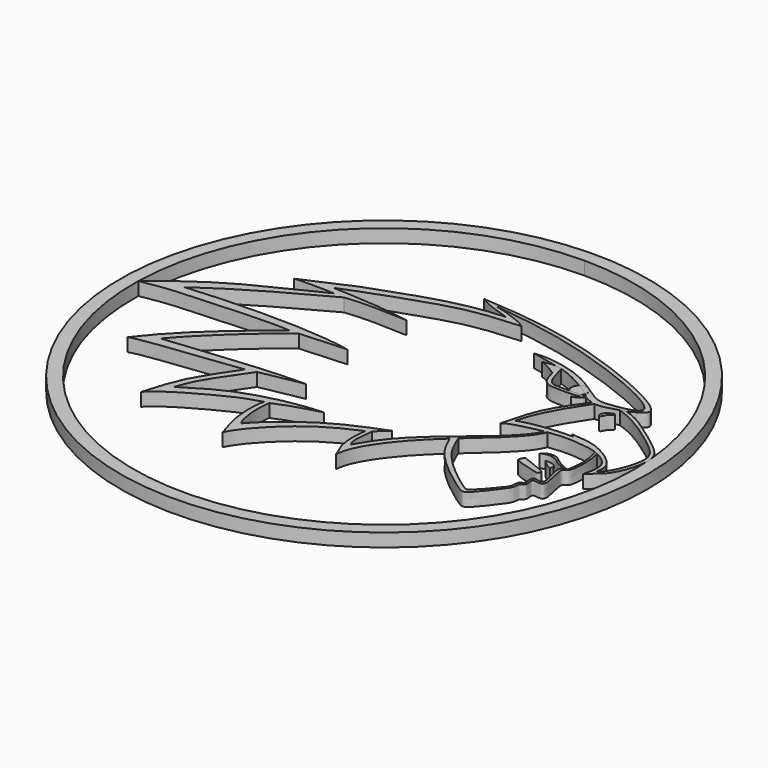
from build123d import *

# Parameters (mm, degrees)
F0_R     = 20
F1_DEPTH = 1
F3_DEPTH = 1
F4_DEPTH = 1
F5_DEPTH = 1


with BuildPart() as f1:
    # F0 (on Top) → F1 (new body)
    with BuildSketch(Plane.XY):
        Circle(F0_R)
        with BuildLine():
            ThreePointArc((0, 19), (13.4350288425, 13.4350288425), (19, 0))
            ThreePointArc((19, 0), (-13.4350288425, -13.4350288425), (0, 19))
        make_face(mode=Mode.SUBTRACT)
    extrude(amount=F1_DEPTH)

    # F0 (on Top) → F5 (cut)
    with BuildSketch(Plane.XY):
        with BuildLine():
            ThreePointArc((2, 17), (1.4142135624, 18.4142135624), (0, 19))
            ThreePointArc((0, 19), (-1.4142135624, 15.5857864376), (2, 17))
        make_face()
    extrude(amount=-F5_DEPTH, mode=Mode.SUBTRACT)


with BuildPart() as f3:
    # F2 (on Top) → F3 (new body)
    with BuildSketch(Plane.XY):
        with BuildLine():
            add(Edge.make_bspline(
                [(-0.4861813504, 11.1744105816), (-0.8512394251, 11.2638310445), (-1.2162974998, 11.3648650216), (-1.5813555744, 11.4542854845)],
                knots=[0, 0, 0, 0, 1.1303700908, 1.1303700908, 1.1303700908, 1.1303700908], degree=3))
            add(Edge.make_bspline(
                [(0.8560517081, 10.4542854845), (0.456931297, 10.5817613038), (-0.7624425914, 10.952583542), (-1.4454943385, 11.374283212), (-1.5813555744, 11.4542854845)],
                knots=[0, 0, 0, 0, 0.5795811507, 1, 1, 1, 1], degree=3))
            add(Edge.make_bspline(
                [(0.8560517081, 10.4542854845), (1.347997395, 10.3436817245), (1.8399430819, 10.2214644504), (2.3318887688, 10.1108606905)],
                knots=[0, 0, 0, 0, 1.5152675074, 1.5152675074, 1.5152675074, 1.5152675074], degree=3))
            add(Edge.make_bspline(
                [(-0.4861813504, 11.1744105816), (-0.0018532867, 11.0755696507), (0.8729949517, 10.8262661766), (2.0316981245, 10.3485118598), (2.3318887688, 10.1108606905)],
                knots=[0, 0, 0, 0, 0.493621531, 1, 1, 1, 1], degree=3))
        make_face()
        with BuildLine():
            add(Edge.make_bspline(
                [(-1.5813555744, 11.4542854845), (1.5137201983, 11.2728479022), (6.8353273779, 10.7000799716), (16.282658027, 6.5869668115), (14.7493827743, 5.8416786773), (14.0054317054, 5.4542854845)],
                knots=[0, 0, 0, 0, 0.4314987059, 0.832199816, 1, 1, 1, 1], degree=3))
            add(Edge.make_bspline(
                [(-0.4861813504, 11.1744105816), (-0.8512394251, 11.2638310445), (-1.2162974998, 11.3648650216), (-1.5813555744, 11.4542854845)],
                knots=[0, 0, 0, 0, 1.1303700908, 1.1303700908, 1.1303700908, 1.1303700908], degree=3))
            add(Edge.make_bspline(
                [(10.5331156468, 6.2760727313), (10.9363930891, 6.0023009623), (11.7608523883, 5.4283523122), (12.6827028969, 5.4977681276), (16.7129876566, 6.1384112415), (6.8471463505, 10.2922851198), (1.9949780392, 10.875952097), (-0.4861813504, 11.1744105816)],
                knots=[0.2889714832, 0.2889714832, 0.2889714832, 0.2889714832, 0.356550035, 0.445023231, 0.5537782213, 0.7718242062, 1, 1, 1, 1], degree=3))
            ThreePointArc((10.5331156468, 6.2760727313), (10.598059942, 6.2051560591), (10.6508410154, 6.1247751273))
            add(Edge.make_bspline(
                [(10.6738684154, 6.0779841061), (10.6672557436, 6.094176268), (10.6595213576, 6.1097407497), (10.6508410154, 6.1247751273)],
                knots=[0.5200147082, 0.5200147082, 0.5200147082, 0.5200147082, 0.5949328564, 0.5949328564, 0.5949328564, 0.5949328564], degree=3))
            ThreePointArc((10.6738684154, 6.0779841061), (10.7117232873, 5.9599696048), (10.7245236322, 5.8366952562))
            ThreePointArc((10.7245236322, 5.8366952562), (10.7193272415, 5.7579001655), (10.7038280777, 5.6804699083))
            add(Edge.make_bspline(
                [(10.8788312047, 5.5142322606), (10.8201676346, 5.574270973), (10.7620682332, 5.6292664848), (10.7038280777, 5.6804699083)],
                knots=[0.0457229123, 0.0457229123, 0.0457229123, 0.0457229123, 0.1098488178, 0.1098488178, 0.1098488178, 0.1098488178], degree=3))
            add(Edge.make_bspline(
                [(11.0054317054, 5.3776609224), (10.9627743647, 5.426050984), (10.9206593746, 5.4714235897), (10.8788312047, 5.5142322606)],
                knots=[0, 0, 0, 0, 0.0457229123, 0.0457229123, 0.0457229123, 0.0457229123], degree=3))
            add(Edge.make_bspline(
                [(11.7051415145, 5.0738393329), (11.4780951892, 5.1390461198), (11.2417685069, 5.2580316606), (11.0054317054, 5.3776609224)],
                knots=[0.7086826403, 0.7086826403, 0.7086826403, 0.7086826403, 1, 1, 1, 1], degree=3))
            add(Edge.make_bspline(
                [(11.9165878221, 5.0287558852), (11.845282437, 5.0385221127), (11.7756595929, 5.0535868258), (11.7051415145, 5.0738393329)],
                knots=[0.6182026893, 0.6182026893, 0.6182026893, 0.6182026893, 0.7086826403, 0.7086826403, 0.7086826403, 0.7086826403], degree=3))
            add(Edge.make_bspline(
                [(13.6013078109, 5.3359311645), (13.1590303776, 5.2060413972), (12.4958934367, 5.0161099675), (12.0665284028, 5.0082195145), (11.9165878221, 5.0287558852)],
                knots=[0.0991333359, 0.0991333359, 0.0991333359, 0.0991333359, 0.4279419343, 0.6182026893, 0.6182026893, 0.6182026893, 0.6182026893], degree=3))
            add(Edge.make_bspline(
                [(14.0054317054, 5.4542854845), (13.870013159, 5.4151232081), (13.7346511528, 5.375091959), (13.6013078109, 5.3359311645)],
                knots=[0, 0, 0, 0, 0.0991333359, 0.0991333359, 0.0991333359, 0.0991333359], degree=3))
        make_face()
        with BuildLine():
            add(Edge.make_bspline(
                [(0.8560517081, 10.4542854845), (1.347997395, 10.3436817245), (1.8399430819, 10.2214644504), (2.3318887688, 10.1108606905)],
                knots=[0, 0, 0, 0, 1.5152675074, 1.5152675074, 1.5152675074, 1.5152675074], degree=3))
            add(Edge.make_bspline(
                [(-11.9945682946, 6.4542854845), (-7.4345962177, 8.526844287), (-8.3451825047, 7.8887416654), (-2.5702483782, 10.2993129908), (0.8560517081, 10.4542854845)],
                knots=[0, 0, 0, 0, 0.4547468229, 1, 1, 1, 1], degree=3))
            add(Edge.make_bspline(
                [(-9.437805973, 6.9979857653), (-10.2901514814, 6.812881167), (-11.1422227862, 6.6393900828), (-11.9945682946, 6.4542854845)],
                knots=[0, 0, 0, 0, 2.6139325861, 2.6139325861, 2.6139325861, 2.6139325861], degree=3))
            add(Edge.make_bspline(
                [(2.3318887688, 10.1108606905), (-0.1704881142, 9.9523263052), (-2.4060494059, 9.6797784859), (-8.1382575205, 7.5277293123), (-9.437805973, 6.9979857653)],
                knots=[0, 0, 0, 0, 0.4735027483, 1, 1, 1, 1], degree=3))
        make_face()
        with BuildLine():
            add(Edge.make_bspline(
                [(-9.437805973, 6.9979857653), (-10.2901514814, 6.812881167), (-11.1422227862, 6.6393900828), (-11.9945682946, 6.4542854845)],
                knots=[0, 0, 0, 0, 2.6139325861, 2.6139325861, 2.6139325861, 2.6139325861], degree=3))
            add(Edge.make_bspline(
                [(-8.9945682946, 6.4542854845), (-9.522863819, 6.5246981059), (-10.5059200736, 6.4690749931), (-11.522878056, 6.5247410497), (-11.9945682946, 6.4542854845)],
                knots=[0, 0, 0, 0, 0.5049517599, 1, 1, 1, 1], degree=3))
            add(Edge.make_bspline(
                [(-8.9945682946, 6.4542854845), (-8.6731177195, 6.6260619146), (-8.3893885889, 6.7883952053), (-8.1571784314, 6.9392999329)],
                knots=[0.8832644452, 0.8832644452, 0.8832644452, 0.8832644452, 0.9768557275, 0.9768557275, 0.9768557275, 0.9768557275], degree=3))
            add(Edge.make_bspline(
                [(-9.437805973, 6.9979857653), (-9.0093557743, 6.9800113372), (-8.5810237757, 6.961155761), (-8.1571784314, 6.9392999329)],
                knots=[0, 0, 0, 0, 0.2013781125, 0.2013781125, 0.2013781125, 0.2013781125], degree=3))
        make_face()
        with BuildLine():
            add(Edge.make_bspline(
                [(8.0054317054, -3.7966177529), (8.2898260757, -4.4579195652), (8.9864830293, -5.954453675), (12.3731367734, -8.445241894), (13.0448971175, -8.7603817483), (14.3507244814, -7.0162171248), (14.8895712447, -6.3204618643), (14.8316427485, -5.6999043858), (15.3390583018, -5.5833833225), (14.9418943677, -4.6397702822), (16.5155719348, -5.3698795524), (15.4397444171, -2.7507816764), (15.9484559288, -2.6639431284), (16.2027875193, -2.3396313354), (16.315607169, -0.8692905211), (16.0054317054, 0.1406347668)],
                knots=[0, 0, 0, 0, 0.1136450834, 0.2600490499, 0.3147574633, 0.4174522444, 0.4885117772, 0.5392127995, 0.5832283808, 0.6383243772, 0.7002940394, 0.8033734923, 0.8435010515, 0.8846597739, 1, 1, 1, 1], degree=3))
            add(Edge.make_bspline(
                [(16.0054317054, 0.1406347668), (15.9367498392, 0.1718007517), (15.8688348063, 0.2002379525), (15.8029340304, 0.2259659243)],
                knots=[0.4452926582, 0.4452926582, 0.4452926582, 0.4452926582, 0.4779376445, 0.4779376445, 0.4779376445, 0.4779376445], degree=3))
            add(Edge.make_bspline(
                [(15.8029340304, 0.2259659243), (16.2024237737, -0.9746317417), (15.9551323563, -2.2067979529), (15.9404590298, -2.6110125574), (15.0831234563, -2.506989592), (16.3334540673, -5.202920191), (14.7459589034, -4.3609787848), (15.182756689, -5.52586244), (14.6262803986, -5.5528238801), (14.7014389749, -6.2739442536), (14.218752005, -6.8356427806), (12.9818490478, -8.3183182278), (12.5435282655, -8.1735127931), (9.1793074854, -5.6536294015), (8.6788500191, -4.1321049701), (8.3839511499, -3.4548977856)],
                knots=[0, 0, 0, 0, 0.1175921657, 0.15453459, 0.2023489346, 0.3052264197, 0.3669995163, 0.4294490254, 0.4729888417, 0.5279170689, 0.5950656627, 0.6938101081, 0.7380707945, 0.8845600614, 1, 1, 1, 1], degree=3))
            add(Edge.make_bspline(
                [(8.0054317054, -3.7966177529), (8.1296512313, -3.683389836), (8.2557395049, -3.5697052226), (8.3839511499, -3.4548977856)],
                knots=[0.5563520178, 0.5563520178, 0.5563520178, 0.5563520178, 0.5948635796, 0.5948635796, 0.5948635796, 0.5948635796], degree=3))
        make_face()
        with BuildLine():
            add(Edge.make_bspline(
                [(-8.9945682946, 6.4542854845), (-8.7218330893, 6.449932218), (-8.4493720874, 6.4339654374), (-8.1766368821, 6.4296121709)],
                knots=[0, 0, 0, 0, 0.8183034693, 0.8183034693, 0.8183034693, 0.8183034693], degree=3))
            add(Edge.make_bspline(
                [(-18.9945682946, 0.4542854845), (-17.5820769946, 1.6270596143), (-14.9381944818, 3.712481166), (-10.3753502253, 5.7164246461), (-8.9945682946, 6.4542854845)],
                knots=[0, 0, 0, 0, 0.4812457167, 0.8832644452, 0.8832644452, 0.8832644452, 0.8832644452], degree=3))
            add(Edge.make_bspline(
                [(-16.3652878255, 1.5516962158), (-17.2418060497, 1.1820214673), (-18.1180500704, 0.8239602329), (-18.9945682946, 0.4542854845)],
                knots=[0, 0, 0, 0, 2.8491097028, 2.8491097028, 2.8491097028, 2.8491097028], degree=3))
            add(Edge.make_bspline(
                [(-8.1766368821, 6.4296121709), (-10.0553413983, 5.4250495729), (-13.461796709, 3.559962101), (-15.4947216945, 2.1565062864), (-16.3652878255, 1.5516962158)],
                knots=[0, 0, 0, 0, 0.571381465, 1, 1, 1, 1], degree=3))
        make_face()
        with BuildLine():
            add(Edge.make_bspline(
                [(-8.9945682946, 6.4542854845), (-8.6731177195, 6.6260619146), (-8.3893885889, 6.7883952053), (-8.1571784314, 6.9392999329)],
                knots=[0.8832644452, 0.8832644452, 0.8832644452, 0.8832644452, 0.9768557275, 0.9768557275, 0.9768557275, 0.9768557275], degree=3))
            add(Edge.make_bspline(
                [(-8.9945682946, 6.4542854845), (-8.7218330893, 6.449932218), (-8.4493720874, 6.4339654374), (-8.1766368821, 6.4296121709)],
                knots=[0, 0, 0, 0, 0.8183034693, 0.8183034693, 0.8183034693, 0.8183034693], degree=3))
            add(Edge.make_bspline(
                [(-3.4766462632, 6.4542854845), (-4.6195402835, 6.4695514404), (-6.0055352159, 6.5970560183), (-7.7097012988, 6.4793692594), (-8.1766368821, 6.4296121709)],
                knots=[0, 0, 0, 0, 0.5412758456, 1, 1, 1, 1], degree=3))
            add(Edge.make_bspline(
                [(-8.1571784314, 6.9392999329), (-7.4818547596, 6.9044764808), (-5.8293263125, 6.7988430674), (-4.3568301948, 6.5929209284), (-3.4766462632, 6.4542854845)],
                knots=[0.2013781125, 0.2013781125, 0.2013781125, 0.2013781125, 0.5222390306, 1, 1, 1, 1], degree=3))
        make_face()
        with BuildLine():
            add(Edge.make_bspline(
                [(4.0054317054, -9.5457145155), (4.0638649507, -8.4116041204), (5.625733879, -6.0741491978), (7.257763763, -4.4781280309), (8.0054317054, -3.7966177529)],
                knots=[0, 0, 0, 0, 0.3245538369, 0.5563520178, 0.5563520178, 0.5563520178, 0.5563520178], degree=3))
            add(Edge.make_bspline(
                [(8.0054317054, -3.7966177529), (8.1296512313, -3.683389836), (8.2557395049, -3.5697052226), (8.3839511499, -3.4548977856)],
                knots=[0.5563520178, 0.5563520178, 0.5563520178, 0.5563520178, 0.5948635796, 0.5948635796, 0.5948635796, 0.5948635796], degree=3))
            add(Edge.make_bspline(
                [(8.3839511499, -3.4548977856), (8.6119808755, -3.2507079994), (10.000478352, -2.0219412426), (11.6740809916, -0.5378026081), (12.0054317054, 0.4542854845)],
                knots=[0.5948635796, 0.5948635796, 0.5948635796, 0.5948635796, 0.6633579887, 1, 1, 1, 1], degree=3))
            add(Edge.make_bspline(
                [(11.8061914617, 0.4261335079), (11.8714310217, 0.4352130962), (11.9401921454, 0.4452058962), (12.0054317054, 0.4542854845)],
                knots=[0, 0, 0, 0, 0.2012193045, 0.2012193045, 0.2012193045, 0.2012193045], degree=3))
            add(Edge.make_bspline(
                [(3.9102742448, -8.0432752147), (4.3586203883, -7.2255821847), (5.5035189512, -5.509628462), (8.568807325, -2.9394624212), (11.3308339869, -0.6975460271), (11.8061914617, 0.4261335079)],
                knots=[0, 0, 0, 0, 0.2887268362, 0.6364737286, 1, 1, 1, 1], degree=3))
            add(Edge.make_bspline(
                [(3.8548011798, -5.9568551369), (3.772172657, -6.5835202766), (3.644234835, -7.5538168559), (3.8406969894, -7.9152672279), (3.9102742448, -8.0432752147)],
                knots=[0, 0, 0, 0, 0.6458490662, 1, 1, 1, 1], degree=3))
            add(Edge.make_bspline(
                [(3.5054317054, -6.1596883461), (3.621979598, -6.0920772764), (3.7382532872, -6.0244662066), (3.8548011798, -5.9568551369)],
                knots=[0, 0, 0, 0, 0.4039806189, 0.4039806189, 0.4039806189, 0.4039806189], degree=3))
            add(Edge.make_bspline(
                [(3.5054317054, -6.1596883461), (3.3600492324, -6.9077194143), (3.4440765238, -8.5284621452), (3.7725241594, -8.9077682238), (4.0054317054, -9.5457145155)],
                knots=[0, 0, 0, 0, 0.5652533657, 1, 1, 1, 1], degree=3))
        make_face()
        with BuildLine():
            add(Edge.make_bspline(
                [(-16.3652878255, 1.5516962158), (-17.2418060497, 1.1820214673), (-18.1180500704, 0.8239602329), (-18.9945682946, 0.4542854845)],
                knots=[0, 0, 0, 0, 2.8491097028, 2.8491097028, 2.8491097028, 2.8491097028], degree=3))
            add(Edge.make_bspline(
                [(-7.9945682946, 1.1069288947), (-9.4194089141, 1.2375310125), (-13.8746096233, 0.9432780806), (-17.3497294719, 0.8182465619), (-18.9945682946, 0.4542854845)],
                knots=[0, 0, 0, 0, 0.5086782206, 1, 1, 1, 1], degree=3))
            add(Edge.make_bspline(
                [(-7.9945682946, 1.1069288947), (-7.7785906263, 1.118545444), (-7.5628871615, 1.1301619933), (-7.3469094932, 1.1417785427)],
                knots=[0, 0, 0, 0, 0.64859573, 0.64859573, 0.64859573, 0.64859573], degree=3))
            add(Edge.make_bspline(
                [(-3.8513934705, 1.3500220375), (-5.0165654781, 1.2806075392), (-6.1817374857, 1.2111930409), (-7.3469094932, 1.1417785427)],
                knots=[0, 0, 0, 0, 3.501713526, 3.501713526, 3.501713526, 3.501713526], degree=3))
            add(Edge.make_bspline(
                [(-16.3652878255, 1.5516962158), (-15.565707993, 1.6230606445), (-13.3888340962, 1.8009877733), (-6.9601712748, 1.95987802), (-3.8513934705, 1.3500220375)],
                knots=[0, 0, 0, 0, 0.3529099079, 1, 1, 1, 1], degree=3))
        make_face()
        with BuildLine():
            add(Edge.make_bspline(
                [(11.8061914617, 0.4261335079), (11.8714310217, 0.4352130962), (11.9401921454, 0.4452058962), (12.0054317054, 0.4542854845)],
                knots=[0, 0, 0, 0, 0.2012193045, 0.2012193045, 0.2012193045, 0.2012193045], degree=3))
            add(Edge.make_bspline(
                [(12.0054317054, 0.4542854845), (11.9335014994, 0.4445855578), (11.8673594997, 0.4352227415), (11.8061914617, 0.4261335079)],
                knots=[0, 0, 0, 0, 0.045093961, 0.045093961, 0.045093961, 0.045093961], degree=3))
        make_face()
        with BuildLine():
            add(Edge.make_bspline(
                [(11.0054317054, 5.3776609224), (10.9766799448, 5.3499652873), (10.9479141187, 5.3222718507), (10.9191216825, 5.2950319835)],
                knots=[0, 0, 0, 0, 0.1163217921, 0.1163217921, 0.1163217921, 0.1163217921], degree=3))
            add(Edge.make_bspline(
                [(11.0054317054, 5.3776609224), (10.9627743647, 5.426050984), (10.9206593746, 5.4714235897), (10.8788312047, 5.5142322606)],
                knots=[0, 0, 0, 0, 0.0457229123, 0.0457229123, 0.0457229123, 0.0457229123], degree=3))
            add(Edge.make_bspline(
                [(10.7124977644, 5.2431622291), (10.7777652371, 5.3272816281), (10.8283263206, 5.4207825248), (10.8788312047, 5.5142322606)],
                knots=[0.6307995672, 0.6307995672, 0.6307995672, 0.6307995672, 1, 1, 1, 1], degree=3))
            add(Edge.make_bspline(
                [(10.7124977709, 5.2431622168), (10.7998791803, 5.2586422167), (10.8707298047, 5.2772768221), (10.9122089251, 5.2919671976), (10.9191216825, 5.2950319835)],
                knots=[0.8539044223, 0.8539044223, 0.8539044223, 0.8539044223, 0.9271251416, 0.9427547052, 0.9427547052, 0.9427547052, 0.9427547052], degree=3))
        make_face()
        with BuildLine():
            add(Edge.make_bspline(
                [(-7.9945682946, 1.1069288947), (-7.7785906263, 1.118545444), (-7.5628871615, 1.1301619933), (-7.3469094932, 1.1417785427)],
                knots=[0, 0, 0, 0, 0.64859573, 0.64859573, 0.64859573, 0.64859573], degree=3))
            add(Edge.make_bspline(
                [(-14.9945682946, -5.5457145155), (-13.7942167508, -3.9619471346), (-11.3654715918, -1.5600629206), (-8.5238978454, 0.7571385041), (-7.9945682946, 1.1069288947)],
                knots=[0, 0, 0, 0, 0.5502062106, 1, 1, 1, 1], degree=3))
            add(Edge.make_bspline(
                [(-13.3645571768, -4.4584060088), (-13.9079856172, -4.8247133491), (-14.4511398542, -5.1794071752), (-14.9945682946, -5.5457145155)],
                knots=[0, 0, 0, 0, 1.9593815435, 1.9593815435, 1.9593815435, 1.9593815435], degree=3))
            add(Edge.make_bspline(
                [(-7.3469094932, 1.1417785427), (-8.4448163694, 0.338849624), (-10.428148874, -1.3877723247), (-12.459579288, -3.3913620914), (-13.3645571768, -4.4584060088)],
                knots=[0, 0, 0, 0, 0.4931522989, 1, 1, 1, 1], degree=3))
        make_face()
        with BuildLine():
            add(Edge.make_bspline(
                [(3.5054317054, -6.1596883461), (1.5487303991, -6.9704932358), (-0.6712385557, -8.5041214516), (-2.5806113885, -10.6743746923), (-2.9945682946, -11.5457145155)],
                knots=[0, 0, 0, 0, 0.5457931521, 1, 1, 1, 1], degree=3))
            add(Edge.make_bspline(
                [(3.5054317054, -6.1596883461), (3.621979598, -6.0920772764), (3.7382532872, -6.0244662066), (3.8548011798, -5.9568551369)],
                knots=[0, 0, 0, 0, 0.4039806189, 0.4039806189, 0.4039806189, 0.4039806189], degree=3))
            add(Edge.make_bspline(
                [(4.7053410672, -5.1438389346), (4.1925152764, -5.5566010997), (4.1383144756, -5.6858497361), (3.8548011798, -5.9568551369)],
                knots=[0, 0, 0, 0, 1.1766109999, 1.1766109999, 1.1766109999, 1.1766109999], degree=3))
            add(Edge.make_bspline(
                [(-2.8363403399, -9.9698845297), (-2.2336621248, -9.1870753445), (0.8172660509, -6.603215349), (3.4794982093, -5.6316746926), (4.7053410672, -5.1438389346)],
                knots=[0, 0, 0, 0, 0.5101161446, 1, 1, 1, 1], degree=3))
            add(Edge.make_bspline(
                [(-2.8363403399, -9.9698845297), (-2.8891743926, -10.499032363), (-2.9417342419, -11.0165666822), (-2.9945682946, -11.5457145155)],
                knots=[0, 0, 0, 0, 1.5837538413, 1.5837538413, 1.5837538413, 1.5837538413], degree=3))
        make_face()
        with BuildLine():
            add(Edge.make_bspline(
                [(10.7124977644, 5.2431622291), (10.7777652371, 5.3272816281), (10.8283263206, 5.4207825248), (10.8788312047, 5.5142322606)],
                knots=[0.6307995672, 0.6307995672, 0.6307995672, 0.6307995672, 1, 1, 1, 1], degree=3))
            add(Edge.make_bspline(
                [(10.5876416139, 5.4552221444), (10.7119645185, 5.4687768368), (10.8132918157, 5.4878681461), (10.8788312047, 5.5142322606)],
                knots=[0.9288619991, 0.9288619991, 0.9288619991, 0.9288619991, 1, 1, 1, 1], degree=3))
            ThreePointArc((10.5876416139, 5.4552221444), (10.1438012047, 5.2370050235), (9.6868620587, 5.4262657895))
            add(Edge.make_bspline(
                [(7.5738726935, 7.3075284909), (7.7347322981, 6.7586938275), (7.9656803002, 5.8009274562), (8.4150621486, 5.4503047461), (8.6410366658, 5.4554705102), (9.3331242163, 5.4294502953), (9.6868620587, 5.4262657895)],
                knots=[0, 0, 0, 0, 0.3157224798, 0.4831189611, 0.6370585107, 0.7892793039, 0.7892793039, 0.7892793039, 0.7892793039], degree=3))
            add(Edge.make_bspline(
                [(7.0054317054, 7.4275257448), (7.194069466, 7.3880026642), (7.3852349329, 7.3470515716), (7.5738726935, 7.3075284909)],
                knots=[0, 0, 0, 0, 0.580968586, 0.580968586, 0.580968586, 0.580968586], degree=3))
            add(Edge.make_bspline(
                [(7.0054317054, 7.4275257448), (7.2368354843, 7.1370684847), (7.3778157625, 6.8481811321), (7.4760666909, 6.5864642458)],
                knots=[0, 0, 0, 0, 0.1150398825, 0.1150398825, 0.1150398825, 0.1150398825], degree=3))
            add(Edge.make_bspline(
                [(7.4760666909, 6.5864642458), (7.599966357, 6.2564252799), (7.7053925655, 5.7159426733), (8.0092209539, 5.4106039251), (8.4152137506, 5.1149664465), (10.1482575277, 5.1607333366), (10.6449614819, 5.231197867), (10.7124977709, 5.2431622168)],
                knots=[0.1150398825, 0.1150398825, 0.1150398825, 0.1150398825, 0.260111316, 0.3884015219, 0.5226464923, 0.7973128006, 0.8539044223, 0.8539044223, 0.8539044223, 0.8539044223], degree=3))
        make_face()
        with BuildLine():
            add(Edge.make_bspline(
                [(10.9191216825, 5.2950319835), (10.8134794781, 5.1950863031), (10.594006189, 5.0007919325), (10.3703408449, 4.9282521033), (10.2546671405, 4.8907813616)],
                knots=[0.1163217921, 0.1163217921, 0.1163217921, 0.1163217921, 0.5431175817, 1, 1, 1, 1], degree=3))
            add(Edge.make_bspline(
                [(10.7124977709, 5.2431622168), (10.7998791803, 5.2586422167), (10.8707298047, 5.2772768221), (10.9122089251, 5.2919671976), (10.9191216825, 5.2950319835)],
                knots=[0.8539044223, 0.8539044223, 0.8539044223, 0.8539044223, 0.9271251416, 0.9427547052, 0.9427547052, 0.9427547052, 0.9427547052], degree=3))
            add(Edge.make_bspline(
                [(10.2546671405, 4.8907813616), (10.3986719378, 4.975685716), (10.5736476202, 5.078847567), (10.6927595619, 5.2177228231), (10.7124977644, 5.2431622291)],
                knots=[0, 0, 0, 0, 0.5191458962, 0.6307995672, 0.6307995672, 0.6307995672, 0.6307995672], degree=3))
        make_face()
        with BuildLine():
            add(Edge.make_bspline(
                [(-13.3645571768, -4.4584060088), (-13.9079856172, -4.8247133491), (-14.4511398542, -5.1794071752), (-14.9945682946, -5.5457145155)],
                knots=[0, 0, 0, 0, 1.9593815435, 1.9593815435, 1.9593815435, 1.9593815435], degree=3))
            add(Edge.make_bspline(
                [(-6.9945682946, -4.4383769855), (-8.0952446112, -4.5501292764), (-8.9275713262, -4.7217926342), (-14.1717169651, -5.2607768412), (-14.9945682946, -5.5457145155)],
                knots=[0, 0, 0, 0, 0.4007034114, 1, 1, 1, 1], degree=3))
            add(Edge.make_bspline(
                [(-6.9945682946, -4.4383769855), (-6.7417011949, -4.3755271472), (-6.4891082987, -4.3126773089), (-6.2362411991, -4.2498274706)],
                knots=[0, 0, 0, 0, 0.7814159605, 0.7814159605, 0.7814159605, 0.7814159605], degree=3))
            add(Edge.make_bspline(
                [(-3.0233417638, -3.6399713717), (-4.0005971612, -3.8386157244), (-5.4580878496, -4.0878689765), (-6.0480198511, -4.2227470447), (-6.2362411991, -4.2498274706)],
                knots=[0, 0, 0, 0, 0.6546808205, 1, 1, 1, 1], degree=3))
            add(Edge.make_bspline(
                [(-13.3645571768, -4.4584060088), (-12.0681423322, -4.3195819823), (-9.1183843322, -4.0484323098), (-5.700757727, -3.6697206087), (-3.0233417638, -3.6399713717)],
                knots=[0, 0, 0, 0, 0.443130057, 1, 1, 1, 1], degree=3))
        make_face()
        with BuildLine():
            add(Edge.make_bspline(
                [(7.0054317054, 7.4275257448), (7.2368354843, 7.1370684847), (7.3778157625, 6.8481811321), (7.4760666909, 6.5864642458)],
                knots=[0, 0, 0, 0, 0.1150398825, 0.1150398825, 0.1150398825, 0.1150398825], degree=3))
            add(Edge.make_bspline(
                [(7.0054317054, 7.4275257448), (6.8482430912, 7.4322433848), (6.5264679528, 7.366887835), (6.3056031438, 7.3433695864), (6.1365221627, 7.2932951152)],
                knots=[0, 0, 0, 0, 0.5135861035, 1, 1, 1, 1], degree=3))
            add(Edge.make_bspline(
                [(7.4760666909, 6.5864642458), (7.274778729, 6.7258843904), (6.8582364553, 6.9873642083), (6.3467408301, 7.2284157521), (6.1365221627, 7.2932951152)],
                knots=[0, 0, 0, 0, 0.497400116, 1, 1, 1, 1], degree=3))
        make_face()
        with BuildLine():
            add(Edge.make_bspline(
                [(-2.9945682946, -11.5457145155), (-3.3689202357, -10.3055201547), (-3.5591313608, -9.9481934959), (-3.7298772911, -7.5308918058), (-3.4945682946, -6.9626686163)],
                knots=[0, 0, 0, 0, 0.4782437861, 1, 1, 1, 1], degree=3))
            add(Edge.make_bspline(
                [(-2.8363403399, -9.9698845297), (-2.8891743926, -10.499032363), (-2.9417342419, -11.0165666822), (-2.9945682946, -11.5457145155)],
                knots=[0, 0, 0, 0, 1.5837538413, 1.5837538413, 1.5837538413, 1.5837538413], degree=3))
            add(Edge.make_bspline(
                [(-3.1803087331, -6.8991845474), (-3.3214866512, -7.8015294341), (-3.1952766606, -9.0527440799), (-3.0059898672, -9.7746249419), (-2.8363403399, -9.9698845297)],
                knots=[0, 0, 0, 0, 0.6138067856, 1, 1, 1, 1], degree=3))
            add(Edge.make_bspline(
                [(-3.1803087331, -6.8991845474), (-3.2851533214, -6.9203459037), (-3.3897237063, -6.94150726), (-3.4945682946, -6.9626686163)],
                knots=[0, 0, 0, 0, 0.3206077026, 0.3206077026, 0.3206077026, 0.3206077026], degree=3))
        make_face()
        with BuildLine():
            add(Edge.make_bspline(
                [(-6.9945682946, -4.4383769855), (-6.7417011949, -4.3755271472), (-6.4891082987, -4.3126773089), (-6.2362411991, -4.2498274706)],
                knots=[0, 0, 0, 0, 0.7814159605, 0.7814159605, 0.7814159605, 0.7814159605], degree=3))
            add(Edge.make_bspline(
                [(-9.9945682946, -10.5457145155), (-9.3742100362, -8.2656466412), (-8.5672696572, -6.8336822299), (-7.3733678919, -4.9657303608), (-6.9945682946, -4.4383769855)],
                knots=[0, 0, 0, 0, 0.5732793336, 1, 1, 1, 1], degree=3))
            add(Edge.make_bspline(
                [(-8.8671809062, -8.8074477389), (-9.2430681035, -9.3907411692), (-9.6186810973, -9.9624210853), (-9.9945682946, -10.5457145155)],
                knots=[0, 0, 0, 0, 2.071852724, 2.071852724, 2.071852724, 2.071852724], degree=3))
            add(Edge.make_bspline(
                [(-6.2362411991, -4.2498274706), (-6.8336737535, -5.1070575407), (-8.3886130268, -7.3405128695), (-8.6195366457, -8.135269396), (-8.8671809062, -8.8074477389)],
                knots=[0, 0, 0, 0, 0.5932918079, 1, 1, 1, 1], degree=3))
        make_face()
        with BuildLine():
            add(Edge.make_bspline(
                [(-3.4945682946, -6.9626686163), (-4.6173458717, -7.3434256483), (-4.6443966723, -7.2185484114), (-9.3685322308, -9.6588319229), (-9.9945682946, -10.5457145155)],
                knots=[0, 0, 0, 0, 0.3681994241, 1, 1, 1, 1], degree=3))
            add(Edge.make_bspline(
                [(-3.1803087331, -6.8991845474), (-3.2851533214, -6.9203459037), (-3.3897237063, -6.94150726), (-3.4945682946, -6.9626686163)],
                knots=[0, 0, 0, 0, 0.3206077026, 0.3206077026, 0.3206077026, 0.3206077026], degree=3))
            add(Edge.make_bspline(
                [(0.0970787078, -5.8130566031), (-0.4660853592, -5.9673427604), (-1.0216870143, -6.1379982253), (-2.0933459666, -6.4298141805), (-3.1803087331, -6.8991845474)],
                knots=[0, 0, 0, 0, 0.4152091703, 1, 1, 1, 1], degree=3))
            add(Edge.make_bspline(
                [(-8.8671809062, -8.8074477389), (-7.8682395965, -8.1962507687), (-5.7447688574, -6.7453350294), (-1.6718116822, -5.8749676682), (0.0970787078, -5.8130566031)],
                knots=[0, 0, 0, 0, 0.4445935625, 1, 1, 1, 1], degree=3))
            add(Edge.make_bspline(
                [(-8.8671809062, -8.8074477389), (-9.2430681035, -9.3907411692), (-9.6186810973, -9.9624210853), (-9.9945682946, -10.5457145155)],
                knots=[0, 0, 0, 0, 2.071852724, 2.071852724, 2.071852724, 2.071852724], degree=3))
        make_face()
    extrude(amount=F3_DEPTH)


with BuildPart() as f3b:
    # F2 (on Top) → F3, piece 2 (new body)
    with BuildSketch(Plane.XY):
        with BuildLine():
            ThreePointArc((9.7532266201, 6.3080109984), (10.0563812755, 6.4328132137), (10.3798798954, 6.379643853))
            add(Edge.make_bspline(
                [(5.0704041496, 7.8671742231), (5.4646223846, 7.8945418861), (6.4589528684, 7.9635709143), (8.7973510038, 7.4072181903), (10.0609980807, 6.5939097333), (10.3798798954, 6.379643853)],
                knots=[0, 0, 0, 0, 0.0906207262, 0.2285712393, 0.2805322177, 0.2805322177, 0.2805322177, 0.2805322177], degree=3))
            add(Edge.make_bspline(
                [(7.0054317054, 7.4275257448), (6.6554511618, 7.5181957443), (5.976492544, 7.6630710228), (5.3660015872, 7.803786557), (5.0704041496, 7.8671742231)],
                knots=[0, 0, 0, 0, 0.5175693137, 1, 1, 1, 1], degree=3))
            add(Edge.make_bspline(
                [(7.5738726935, 7.3075284909), (7.3888925134, 7.3580919747), (7.199122916, 7.3991532482), (7.0054317054, 7.4275257448)],
                knots=[0.8979763037, 0.8979763037, 0.8979763037, 0.8979763037, 1, 1, 1, 1], degree=3))
            add(Edge.make_bspline(
                [(9.7532266201, 6.3080109984), (9.1877875802, 6.6334803408), (8.4324154579, 7.0728497643), (7.5738726935, 7.3075284909)],
                knots=[0.4244568909, 0.4244568909, 0.4244568909, 0.4244568909, 0.8979763037, 0.8979763037, 0.8979763037, 0.8979763037], degree=3))
        make_face()
    extrude(amount=F3_DEPTH)


with BuildPart() as f3c:
    # F2 (on Top) → F3, piece 3 (new body)
    with BuildSketch(Plane.XY):
        with BuildLine():
            ThreePointArc((10.5876416139, 5.4552221444), (10.6577639795, 5.5616412033), (10.7038280777, 5.6804699083))
            add(Edge.make_bspline(
                [(10.7038280777, 5.6804699083), (10.4254276085, 5.9252332853), (10.1363946185, 6.0875095202), (9.7628660978, 6.3024624702), (9.7532266201, 6.3080109984)],
                knots=[0.1098488178, 0.1098488178, 0.1098488178, 0.1098488178, 0.4163844384, 0.4244568909, 0.4244568909, 0.4244568909, 0.4244568909], degree=3))
            ThreePointArc((9.7532266201, 6.3080109984), (9.5262158923, 5.8817268938), (9.6868620587, 5.4262657895))
            add(Edge.make_bspline(
                [(9.6868620587, 5.4262657895), (10.0112308942, 5.4233456767), (10.3437027082, 5.4286259445), (10.5876416139, 5.4552221444)],
                knots=[0.7892793039, 0.7892793039, 0.7892793039, 0.7892793039, 0.9288619991, 0.9288619991, 0.9288619991, 0.9288619991], degree=3))
        make_face()
    extrude(amount=F3_DEPTH)


with BuildPart() as f3d:
    # F2 (on Top) → F3, piece 4 (new body)
    with BuildSketch(Plane.XY):
        with BuildLine():
            add(Edge.make_bspline(
                [(15.0166591629, -3.0328873545), (14.8289271144, -2.977658953), (14.579419011, -2.8200348556), (14.2519401221, -2.5694584846), (14.1962645575, -2.4386267178)],
                knots=[0, 0, 0, 0, 0.5013763221, 1, 1, 1, 1], degree=3))
            add(Edge.make_bspline(
                [(14.1962645575, -2.4386267178), (14.3243505563, -2.474091232), (14.5566133771, -2.4338478117), (14.9673135163, -2.5798806066), (15.0577574353, -2.7866188023), (15.0279821445, -2.9602306806), (15.0166591629, -3.0328873545)],
                knots=[0, 0, 0, 0, 0.2800515295, 0.5692061441, 0.7754675717, 1, 1, 1, 1], degree=3))
        make_face()
    extrude(amount=F3_DEPTH)


with BuildPart() as f3e:
    # F2 (on Top) → F3, piece 5 (new body)
    with BuildSketch(Plane.XY):
        with BuildLine():
            add(Edge.make_bspline(
                [(15.6757831573, -2.5491658598), (15.5804967169, -2.5348730203), (15.5097852205, -2.539949552), (14.8815367571, -2.2217926339), (14.7052041272, -2.0078864536), (14.0075978186, -1.6873081937), (13.5486286244, -1.8547309471), (13.3373988792, -1.951631275)],
                knots=[0, 0, 0, 0, 0.127602772, 0.3560877522, 0.518700647, 0.7575961092, 1, 1, 1, 1], degree=3))
            add(Edge.make_bspline(
                [(15.6757831573, -2.5491658598), (15.7188904445, -2.5599426816), (15.8044281877, -2.5252249278), (15.846827513, -2.5363364068), (15.8858858049, -2.4896676186)],
                knots=[0, 0, 0, 0, 0.5236012195, 1, 1, 1, 1], degree=3))
            add(Edge.make_bspline(
                [(13.3373988792, -1.951631275), (13.4808437724, -1.7994007422), (13.8393374483, -1.5966043948), (14.3073780775, -1.6344663908), (14.5813395519, -1.744710437), (15.0536914932, -2.1938165325), (15.5297726614, -2.3750418621), (15.7848894108, -2.518583576), (15.8858858049, -2.4896676186)],
                knots=[0, 0, 0, 0, 0.1901490461, 0.3512654216, 0.4825183776, 0.6763356784, 0.8558883201, 1, 1, 1, 1], degree=3))
        make_face()
    extrude(amount=F3_DEPTH)


with BuildPart() as f3f:
    # F2 (on Top) → F3, piece 6 (new body)
    with BuildSketch(Plane.XY):
        with BuildLine():
            add(Edge.make_bspline(
                [(14.5235862583, -3.9308825508), (14.1481318445, -3.8389207533), (12.9666371586, -3.5181886782), (12.8219016087, -3.3438601917), (12.8980182445, -3.2009991292), (12.954743021, -2.9864790438), (13.0803828469, -2.9221494616), (13.2149860237, -3.0091750226), (14.6793113647, -3.5718388249), (14.8619141768, -3.6418550318), (14.9184337185, -3.7602676441), (14.8432189314, -3.9376521646), (14.7760719976, -3.9870009769), (14.6749975062, -3.9679684126), (14.5235862583, -3.9308825508)],
                knots=[0, 0, 0, 0, 0.1965348484, 0.2609912403, 0.318742608, 0.3915515062, 0.4415614166, 0.5030473002, 0.6964541821, 0.7664396, 0.8159812122, 0.8818077175, 0.9207424775, 1, 1, 1, 1], degree=3))
        make_face()
    extrude(amount=F3_DEPTH)


with BuildPart() as f3g:
    # F2 (on Top) → F3, piece 7 (new body)
    with BuildSketch(Plane.XY):
        with BuildLine():
            add(Edge.make_bspline(
                [(13.6758415028, 4.7596092336), (13.5967514361, 4.7994285712), (13.1085024743, 4.5628672925), (12.9487815042, 4.1578801595), (13.2075850142, 3.8624631227), (13.3992486383, 4.5425383048), (13.7117965258, 4.612714891), (13.7098446564, 4.7424897253), (13.6758415028, 4.7596092336)],
                knots=[0, 0, 0, 0, 0.2147215115, 0.4045126008, 0.5322187037, 0.7487907564, 0.907684886, 1, 1, 1, 1], degree=3))
        make_face()
    extrude(amount=F3_DEPTH)


with BuildPart() as f4:
    # F2 (on Top) → F4 (new body)
    with BuildSketch(Plane.XY):
        with BuildLine():
            ThreePointArc((10.6738684154, 6.0779841061), (10.6628633242, 6.1016299198), (10.6508410154, 6.1247751273))
            add(Edge.make_bspline(
                [(10.6508410154, 6.1247751273), (10.6123614215, 6.1914218944), (10.5552927324, 6.2476515213), (10.4949456982, 6.3019640939)],
                knots=[0.5949328564, 0.5949328564, 0.5949328564, 0.5949328564, 0.9270418741, 0.9270418741, 0.9270418741, 0.9270418741], degree=3))
            add(Edge.make_bspline(
                [(10.3798798954, 6.379643853), (10.4186336391, 6.3536040959), (10.4569906726, 6.3276863418), (10.4949456982, 6.3019640939)],
                knots=[0.2805322177, 0.2805322177, 0.2805322177, 0.2805322177, 0.2868470414, 0.2868470414, 0.2868470414, 0.2868470414], degree=3))
            ThreePointArc((10.3798798954, 6.379643853), (10.0563812755, 6.4328132137), (9.7532266201, 6.3080109984))
            add(Edge.make_bspline(
                [(10.7038280777, 5.6804699083), (10.4254276085, 5.9252332853), (10.1363946185, 6.0875095202), (9.7628660978, 6.3024624702), (9.7532266201, 6.3080109984)],
                knots=[0.1098488178, 0.1098488178, 0.1098488178, 0.1098488178, 0.4163844384, 0.4244568909, 0.4244568909, 0.4244568909, 0.4244568909], degree=3))
            add(Edge.make_bspline(
                [(10.7038280777, 5.6804699083), (10.7116239108, 5.82296017), (10.7197676625, 5.965592616), (10.6738684154, 6.0779841061)],
                knots=[0, 0, 0, 0, 0.5200147082, 0.5200147082, 0.5200147082, 0.5200147082], degree=3))
        make_face()
    extrude(amount=F4_DEPTH)


with BuildPart() as f4b:
    # F2 (on Top) → F4, piece 2 (new body)
    with BuildSketch(Plane.XY):
        with BuildLine():
            ThreePointArc((9.6868620587, 5.4262657895), (10.1438012047, 5.2370050235), (10.5876416139, 5.4552221444))
            add(Edge.make_bspline(
                [(9.6868620587, 5.4262657895), (10.0112308942, 5.4233456767), (10.3437027082, 5.4286259445), (10.5876416139, 5.4552221444)],
                knots=[0.7892793039, 0.7892793039, 0.7892793039, 0.7892793039, 0.9288619991, 0.9288619991, 0.9288619991, 0.9288619991], degree=3))
        make_face()
    extrude(amount=F4_DEPTH)


with BuildPart() as f4c:
    # F2 (on Top) → F4, piece 3 (new body)
    with BuildSketch(Plane.XY):
        with BuildLine():
            add(Edge.make_bspline(
                [(14.0054317054, 5.4542854845), (14.9412901942, 5.1916822992), (16.4010482207, 4.1444433689), (18.0838201897, 2.9411236702), (19.3501702979, 1.646969241), (18.3201688128, -1.5541278268), (17.4757387709, -1.9311968708), (17.0011911541, -2.3996017408)],
                knots=[0, 0, 0, 0, 0.2264998178, 0.4217600106, 0.5944651699, 0.8258545857, 1, 1, 1, 1], degree=3))
            add(Edge.make_bspline(
                [(13.6013078109, 5.3359311645), (13.7349883283, 5.3746632012), (13.871751188, 5.4155534479), (14.0054317054, 5.4542854845)],
                knots=[0, 0, 0, 0, 0.4210984055, 0.4210984055, 0.4210984055, 0.4210984055], degree=3))
            add(Edge.make_bspline(
                [(17.3990372568, -1.7081559636), (17.5657439743, -1.5763406362), (18.0496977944, -1.1868229083), (19.0506415392, 1.4736900604), (18.0181119804, 2.6698101579), (16.0785520186, 4.1309137139), (14.603589737, 4.9959999028), (13.6013078109, 5.3359311645)],
                knots=[0, 0, 0, 0, 0.1290501439, 0.3619698436, 0.5346404203, 0.756019888, 1, 1, 1, 1], degree=3))
            add(Edge.make_bspline(
                [(13.28654401, 1.173744211), (13.7021575486, 1.14398161), (14.5573226113, 1.0827421791), (15.8297851215, 0.7306726294), (17.6387384734, -0.5394287657), (17.4698293329, -1.36299032), (17.3990372568, -1.7081559636)],
                knots=[0, 0, 0, 0, 0.2354516611, 0.4844645707, 0.7839322181, 1, 1, 1, 1], degree=3))
            add(Edge.make_bspline(
                [(13.5917295868, 0.9633864975), (13.4409732972, 1.0335057353), (13.4373002996, 1.1036249731), (13.28654401, 1.173744211)],
                knots=[0, 0, 0, 0, 0.3706596874, 0.3706596874, 0.3706596874, 0.3706596874], degree=3))
            add(Edge.make_bspline(
                [(9.6054519693, 0.4269744677), (9.853664256, 0.5096220348), (10.4562848393, 0.710277392), (12.2357743054, 0.960711834), (13.1596103311, 0.962534129), (13.5917295868, 0.9633864975)],
                knots=[0, 0, 0, 0, 0.2715452004, 0.6592692457, 1, 1, 1, 1], degree=3))
            add(Edge.make_bspline(
                [(11.9165878221, 5.0287558852), (11.3425327774, 4.1788621649), (10.3437300639, 2.5701336631), (9.7693168044, 1.1143182933), (9.6054519693, 0.4269744677)],
                knots=[0, 0, 0, 0, 0.5357507621, 1, 1, 1, 1], degree=3))
            add(Edge.make_bspline(
                [(11.9165878221, 5.0287558852), (11.845282437, 5.0385221127), (11.7756595929, 5.0535868258), (11.7051415145, 5.0738393329)],
                knots=[0.6182026893, 0.6182026893, 0.6182026893, 0.6182026893, 0.7086826403, 0.7086826403, 0.7086826403, 0.7086826403], degree=3))
            add(Edge.make_bspline(
                [(9.1225616634, -0.3920310992), (9.3676293748, 0.603406886), (9.8583032693, 2.5964700695), (11.0890785433, 4.2474456445), (11.7051415145, 5.0738393329)],
                knots=[0, 0, 0, 0, 0.4994512936, 1, 1, 1, 1], degree=3))
            add(Edge.make_bspline(
                [(11.8061914617, 0.4261335079), (11.2357652091, 0.3413713076), (10.9227204108, 0.202924792), (9.4351189338, -0.0785005318), (9.1225616634, -0.3920310992)],
                knots=[0.045093961, 0.045093961, 0.045093961, 0.045093961, 0.465620432, 1, 1, 1, 1], degree=3))
            add(Edge.make_bspline(
                [(12.0054317054, 0.4542854845), (11.9335014994, 0.4445855578), (11.8673594997, 0.4352227415), (11.8061914617, 0.4261335079)],
                knots=[0, 0, 0, 0, 0.045093961, 0.045093961, 0.045093961, 0.045093961], degree=3))
            add(Edge.make_bspline(
                [(15.8029340304, 0.2259659243), (15.7777926889, 0.2357812219), (15.3504022222, 0.3978228375), (14.5701109851, 0.509219344), (13.1618734332, 0.6455609889), (12.0054317054, 0.4542854845)],
                knots=[0.4779376445, 0.4779376445, 0.4779376445, 0.4779376445, 0.4903918035, 0.6921500906, 1, 1, 1, 1], degree=3))
            add(Edge.make_bspline(
                [(16.0054317054, 0.1406347668), (15.9367498392, 0.1718007517), (15.8688348063, 0.2002379525), (15.8029340304, 0.2259659243)],
                knots=[0.4452926582, 0.4452926582, 0.4452926582, 0.4452926582, 0.4779376445, 0.4779376445, 0.4779376445, 0.4779376445], degree=3))
            add(Edge.make_bspline(
                [(17.0011911541, -2.3996017408), (17.144370672, -1.890038021), (17.4296118398, -0.7055922652), (16.4283507375, -0.0512745232), (16.0054317054, 0.1406347668)],
                knots=[0, 0, 0, 0, 0.2442761926, 0.4452926582, 0.4452926582, 0.4452926582, 0.4452926582], degree=3))
        make_face()
    extrude(amount=F4_DEPTH)


solid = Compound([f1.part, f3.part, f3b.part, f3c.part, f3d.part, f3e.part, f3f.part, f3g.part, f4.part, f4b.part, f4c.part])
